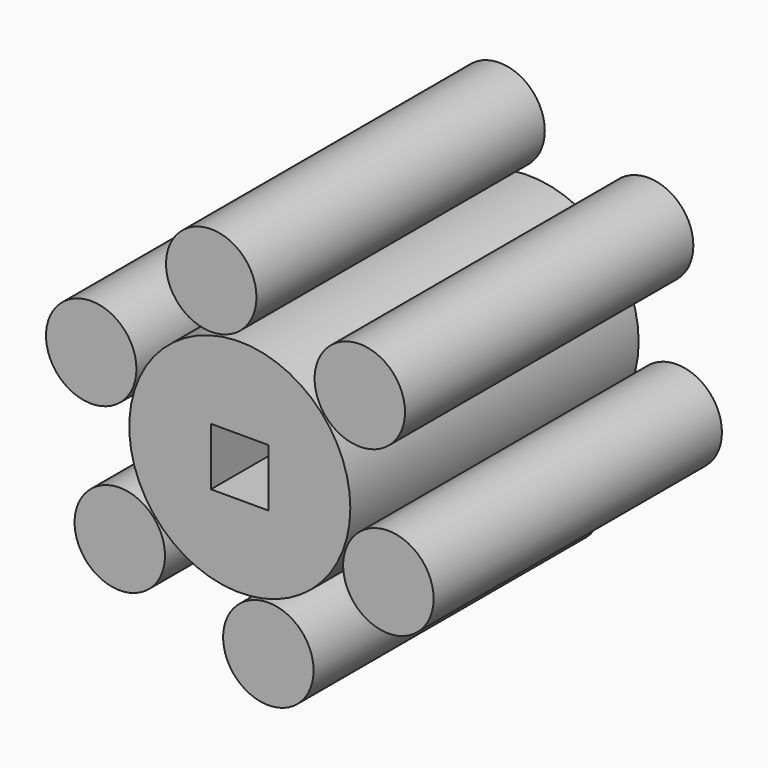
from build123d import *

# Parameters (mm, degrees)
F0_R     = 15.936550819
F1_DEPTH = 63.5
F0_R_2   = 38.9510369052
F0_R_3   = 26.7223642195
F5_DEPTH = 25.4
F8_W     = 20.32
F8_H     = 20.32
F9_DEPTH = 127.001


# Not quite as in the source:
# - the program builds the solid bodies; features that only make, move or delete a surface that nothing else refers to are left out


with BuildPart() as f1:
    # F0 (on Front) → F1 (new body, symmetric)
    with BuildSketch(Plane.XZ):
        with Locations((42.2912457866, 36.0400506581)):
            Circle(F0_R)
    extrude(amount=F1_DEPTH, both=True)

    # F4 (on face) → F5 (cut)
    with BuildSketch(Plane(origin=(23.2564192551, 0, 0), x_dir=(0, -1, 0), z_dir=(-1, 0, 0))):
        Polygon((-131.7048221827, 0), (-70.3143179417, 0), (-70.3143179417, 7.7529181726), (-170.3111678362, 7.7529181726), (-170.3111678362, 0), align=None)
        Polygon((-70.3143179417, -7.7529181726), (-70.3143179417, 0), (-131.7048221827, 0), (-170.3111678362, 0), (-170.3111678362, -7.7529181726), align=None)
    extrude(amount=-F5_DEPTH, mode=Mode.SUBTRACT)


with BuildPart() as f1b:
    # F0 (on Front) → F1, piece 2 (new body, symmetric)
    with BuildSketch(Plane.XZ):
        Circle(F0_R_2)
        Circle(F0_R_3, mode=Mode.SUBTRACT)
        Circle(F0_R_3)
    extrude(amount=F1_DEPTH, both=True)

    # F8 (on face) → F9 (cut, through all)
    with BuildSketch(Plane.XZ.offset(63.5)):
        Rectangle(F8_W, F8_H)
    extrude(amount=-F9_DEPTH, mode=Mode.SUBTRACT)


with BuildPart() as f1c:
    # F0 (on Front) → F1, piece 3 (new body, symmetric)
    with BuildSketch(Plane.XZ):
        with Locations((-10.0659765303, 54.645318538)):
            Circle(F0_R)
    extrude(amount=F1_DEPTH, both=True)


with BuildPart() as f1d:
    # F0 (on Front) → F1, piece 4 (new body, symmetric)
    with BuildSketch(Plane.XZ):
        with Locations((-52.3572223169, 18.6052678798)):
            Circle(F0_R)
    extrude(amount=F1_DEPTH, both=True)


with BuildPart() as f1e:
    # F0 (on Front) → F1, piece 5 (new body, symmetric)
    with BuildSketch(Plane.XZ):
        with Locations((-42.2912457866, -36.0400506581)):
            Circle(F0_R)
    extrude(amount=F1_DEPTH, both=True)


with BuildPart() as f1f:
    # F0 (on Front) → F1, piece 6 (new body, symmetric)
    with BuildSketch(Plane.XZ):
        with Locations((10.0659765303, -54.645318538)):
            Circle(F0_R)
    extrude(amount=F1_DEPTH, both=True)


with BuildPart() as f1g:
    # F0 (on Front) → F1, piece 7 (new body, symmetric)
    with BuildSketch(Plane.XZ):
        with Locations((52.3572223169, -18.6052678798)):
            Circle(F0_R)
    extrude(amount=F1_DEPTH, both=True)


solid = Compound([f1.part, f1b.part, f1c.part, f1d.part, f1e.part, f1f.part, f1g.part])
